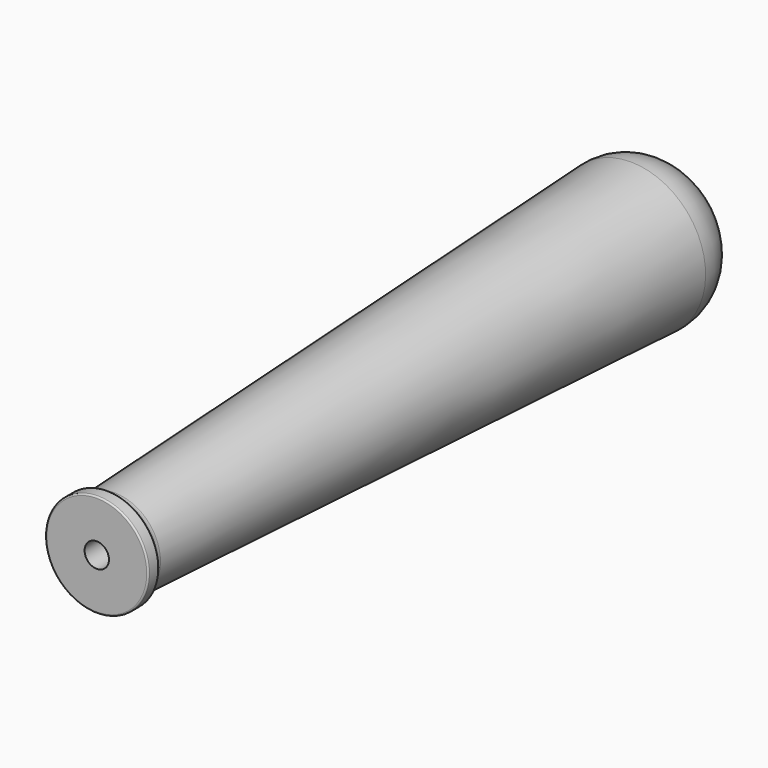
from build123d import *

# Parameters (mm, degrees)
F3_R     = 0.762
F4_R     = 0.762
F5_R     = 25.4
F8_D     = 12
F8_DEPTH = 254
F8_TIP   = 3.6051637142


# Not quite as in the source:
# - a fillet or chamfer that OpenCascade refuses, or shapes differently, is made with other operations: its cross-section is extruded or revolved along the edge and cut away or added


with BuildPart() as f1:
    # F0 (on Right) → F1 (revolve)
    with BuildSketch(Plane.YZ):
        Polygon((-247.65, 25.3958042773), (-254, 25.3958042773), (-254, 0), (101.6, 0), (101.6, 38.1), (-247.65, 22.2208042773), align=None)
    revolve(axis=Axis((0, -76.2, 0), (0, 1, 0)))

    # F2: fillet of radius 5.08 on 1 edges, made by hand

    # F2_s1 → F2_t2 (revolve)
    with BuildSketch(Plane.YZ):
        with BuildLine():
            ThreePointArc((-247.65, 25.3958042773), (-245.6776265029, 23.1782755766), (-242.802840851, 22.4411879247))
            Line((-242.802840851, 22.4411879247), (-242.7982262159, 22.3396927763))
            Line((-242.7982262159, 22.3396927763), (-247.6453853649, 22.119309129))
            Line((-247.6453853649, 22.119309129), (-247.7516, 22.2208042773))
            ThreePointArc((-247.7516, 22.2208042773), (-247.7516, 23.8083042773), (-247.7423285478, 25.353401456))
            Line((-247.7423285478, 25.353401456), (-247.65, 25.3958042773))
        make_face()
    revolve(axis=Axis((0, -247.65, 0), (0, 1, 0)))

    # F3
    f3_edges = [f1.edges().sort_by_distance(p)[0] for p in [
        (0, -254, -25.395804),
    ]]
    fillet(f3_edges, radius=F3_R)

    # F4
    f4_edges = [f1.edges().sort_by_distance(p)[0] for p in [
        (0, -247.65, -25.395804),
    ]]
    fillet(f4_edges, radius=F4_R)

    # F5
    f5_edges = [f1.edges().sort_by_distance(p)[0] for p in [
        (0, 101.6, -38.1),
    ]]
    fillet(f5_edges, radius=F5_R)

    # F8
    with Locations(Plane.XZ.offset(254)):
        with Locations((0, 0)):
            Hole(F8_D / 2, depth=F8_DEPTH)
            with Locations((0, 0, -(F8_DEPTH + F8_TIP / 2))):  # 118° drill point
                Cone(0, F8_D / 2, F8_TIP, mode=Mode.SUBTRACT)


solid = f1.part
